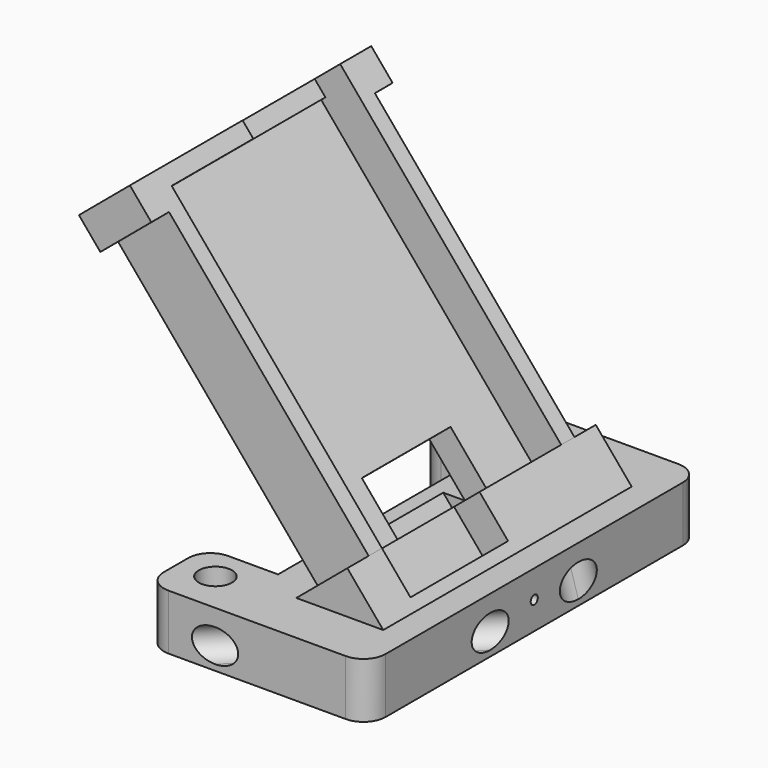
from build123d import *

# Parameters (mm, degrees)
F0_W      = 20
F0_H      = 37.5
F1_DEPTH  = 5
F3_D      = 3
F4_W      = 6.5
F4_H      = 24
F5_DEPTH  = 6
F6_R      = 2
F10_DEPTH = 50
F14_W     = 23.2
F14_H     = 31
F15_DEPTH = 6
F16_W     = 20.2
F16_H     = 30.2
F17_DEPTH = 3.5
F19_DEPTH = 14
F20_W     = 10
F20_H     = 5
F21_DEPTH = 4
F22_W     = 11
F22_H     = 2
F23_DEPTH = 3
F24_W     = 11
F24_H     = 4
F25_DEPTH = 3
F27_DEPTH = 2
F29_DEPTH = 2
F30_R     = 0.4
F31_DEPTH = 70


# Not quite as in the source:
# - a feature names something its author has since deleted; it is built from what else it names


with BuildPart() as f1:
    # F0 (on Top) → F1 (new body)
    with BuildSketch(Plane.XY):
        Rectangle(F0_W, F0_H)
    extrude(amount=F1_DEPTH)

    # F3 (through all)
    with Locations(Plane(origin=(0, 0, 0), x_dir=(1, 0, 0), z_dir=(0, 0, -1))):
        with Locations((-6.75, 15), (-6.75, -15)):
            Hole(F3_D / 2)

    # F4 (on Top) → F5 (cut)
    with BuildSketch(Plane.XY):
        with Locations((-6.75, 0)):
            Rectangle(F4_W, F4_H)
    extrude(amount=F5_DEPTH, mode=Mode.SUBTRACT)

    # F6
    f6_edges = [f1.edges().sort_by_distance(p)[0] for p in [
        (-10, -18.75, 2.5),
        (10, -18.75, 2.5),
        (10, 18.75, 2.5),
        (-10, 18.75, 2.5),
        (-10, -12, 2.5),
        (-10, 12, 2.5),
    ]]
    fillet(f6_edges, radius=F6_R)

    # F9 (on line) → F10 (cut)
    with BuildSketch(Plane(origin=(5.0561841595, -5.0561841595, 0), x_dir=(0.7071067812, 0.7071067812, 0), z_dir=(0.7071067812, -0.7071067812, 0))):
        with BuildLine():
            ThreePointArc((10.5836309448, 0.525), (11.626613447, 0.9570174977), (12.0586309448, 2))
            ThreePointArc((12.0586309448, 2), (9.5406484425, 3.0429825023), (10.5836309448, 0.525))
        make_face()
    extrude(amount=-F10_DEPTH, mode=Mode.SUBTRACT)

    # F11: F1 across plane


with BuildPart() as f1_1:
    add(f1.part)
    add(f1.part.mirror(Plane.XZ), mode=Mode.INTERSECT)

    # F14 (on line) → F15 (join)
    with BuildSketch(Plane(origin=(2.3153133603, 0, 1.9427785867), x_dir=(0, 1, 0), z_dir=(0.7660444431, 0, 0.6427876097))):
        with Locations((0, 19.490919118)):
            Rectangle(F14_W, F14_H)
    extrude(amount=F15_DEPTH)

    # F16 (on face) → F17 (cut)
    with BuildSketch(Plane(origin=(6.911580019, 0, 5.7995042448), x_dir=(0, 1, 0), z_dir=(0.7660444431, 0, 0.6427876097))):
        with Locations((0, 18.390919118)):
            Rectangle(F16_W, F16_H)
    extrude(amount=-F17_DEPTH, mode=Mode.SUBTRACT)

    # F18 (on Front) → F19 (join, symmetric)
    with BuildSketch(Plane.XZ):
        Polygon((4.3462666587, 8.8567256581), (-0.25, 5), (7.582443736, 5), align=None)
    extrude(amount=F19_DEPTH, both=True)

    # F20 (on face) → F21 (cut)
    with BuildSketch(Plane(origin=(4.2304244681, 0, 3.5497476109), x_dir=(0, 1, 0), z_dir=(0.7660444431, 0, 0.6427876097))):
        with Locations((0, 6.490919118)):
            Rectangle(F20_W, F20_H)
    extrude(amount=-F21_DEPTH, mode=Mode.SUBTRACT)

    # F22 (on face) → F23 (cut)
    with BuildSketch(Plane(origin=(6.911580019, 0, 5.7995042448), x_dir=(0, 1, 0), z_dir=(0.7660444431, 0, 0.6427876097))):
        with Locations((4.6, 34.490919118)):
            Rectangle(F22_W, F22_H)
    extrude(amount=-F23_DEPTH, mode=Mode.SUBTRACT)

    # F24 (on face) → F25 (cut)
    with BuildSketch(Plane(origin=(6.911580019, 0, 5.7995042448), x_dir=(0, 1, 0), z_dir=(0.7660444431, 0, 0.6427876097))):
        with Locations((-4.6, 1.990919118)):
            Rectangle(F24_W, F24_H)
    extrude(amount=-F25_DEPTH, mode=Mode.SUBTRACT)

    # F26 (on face) → F27 (join)
    with BuildSketch(Plane.XZ.offset(11.6)):
        Polygon((-15.5801492416, 32.6041033948), (-20.1764159003, 28.7473777367), (-18.2480530712, 26.4492444073), (-13.6517864125, 30.3059700655), align=None)
    extrude(amount=F27_DEPTH)

    # F28 (on face) → F29 (join)
    with BuildSketch(Plane(origin=(0, 11.6, 0), x_dir=(-1, 0, 0), z_dir=(0, 1, 0))):
        Polygon((20.1764159003, 28.7473777367), (15.5801492416, 32.6041033948), (13.6517864125, 30.3059700655), (18.2480530712, 26.4492444073), align=None)
    extrude(amount=F29_DEPTH)

    # F30 (on face) → F31 (cut)
    with BuildSketch(Plane.YZ.offset(10)):
        with Locations((0, 2.5)):
            Circle(F30_R)
    extrude(amount=-F31_DEPTH, mode=Mode.SUBTRACT)


solid = f1_1.part
